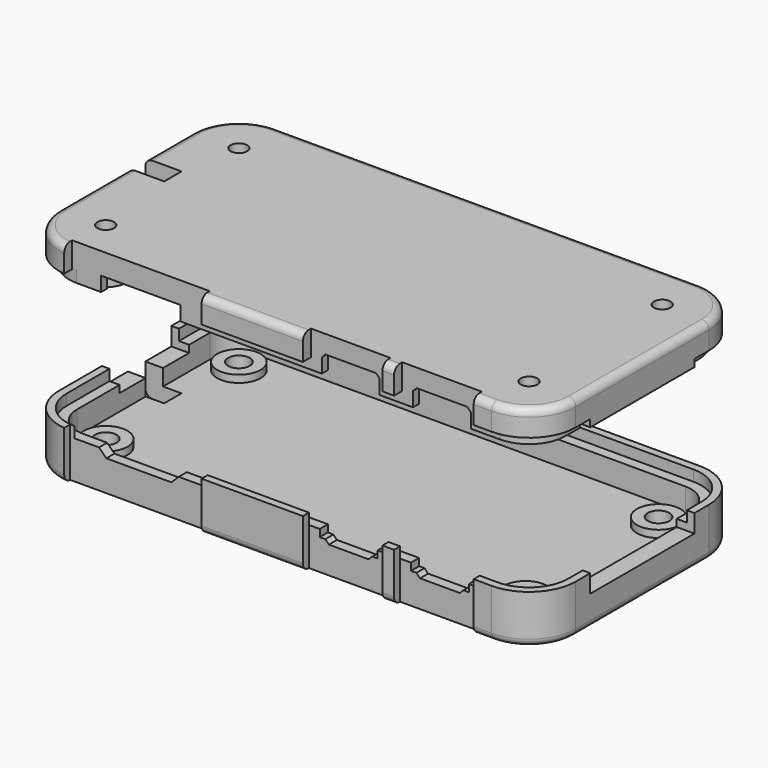
from build123d import *

# Parameters (mm, degrees)
F1_DEPTH  = 2
F2_DEPTH  = 3.25
F3_R      = 3
F4_DEPTH  = 1
F6_W      = 2.45
F6_H      = 12
F6_W_2    = 11
F6_H_2    = 2.45
F6_W_3    = 8
F6_H_3    = 18
F7_DEPTH  = 1
F10_DEPTH = 2
F11_DEPTH = 3
F12_W     = 2.45
F12_H     = 12
F13_DEPTH = 1
F12_W_2   = 11
F12_H_2   = 2.45
F14_DEPTH = 2
F12_W_3   = 8
F15_DEPTH = 2
F12_H_3   = 18
F16_DEPTH = 0.5
F17_R     = 3
F18_DEPTH = 4
F20_D     = 2.3
F20_DEPTH = 13
F20_TIP   = 0.6909897119
F22_D     = 3
F22_DEPTH = 13
F22_TIP   = 0.9012909285
F23_W     = 3
F23_H     = 4.25
F24_DEPTH = 5
F25_W     = 3
F25_H     = 4
F26_DEPTH = 5
F27_R     = 1
F27_2_R   = 1
F28_W     = 5.5
F28_H     = 2.45
F29_DEPTH = 0.5
F30_SIZE  = 0.49999
F31_W     = 7
F31_H     = 2.45
F32_DEPTH = 0.5
F33_SIZE  = 0.49999
F34_W     = 19.5
F34_H     = 1.4
F34_W_2   = 4.6
F35_DEPTH = 1.5
F37_W     = 4.6
F37_H     = 1.05
F37_W_2   = 19.5
F38_DEPTH = 1.5
F39_SIZE  = 1
F40_W     = 11
F40_H     = 3.5
F40_W_2   = 19
F41_DEPTH = 1.4
F42_W     = 11
F42_H     = 6.75
F42_W_2   = 19
F43_DEPTH = 1.05


# Not quite as in the source:
# - a fillet or chamfer is up to 0.001 mm smaller than in the source, because OpenCascade refuses the exact size


with BuildPart() as f1:
    # F0 (on Top) → F1 (new body)
    with BuildSketch(Plane.XY):
        with BuildLine():
            Line((62, 32.95), (3.5, 32.95))
            ThreePointArc((3.5, 32.95), (-1.0608387387, 31.0608387387), (-2.95, 26.5))
            Line((-2.95, 26.5), (-2.95, 3.5))
            ThreePointArc((-2.95, 3.5), (-1.0608387387, -1.0608387387), (3.5, -2.95))
            Line((3.5, -2.95), (62, -2.95))
            ThreePointArc((62, -2.95), (66.5608387387, -1.0608387387), (68.45, 3.5))
            Line((68.45, 3.5), (68.45, 26.5))
            ThreePointArc((68.45, 26.5), (66.5608387387, 31.0608387387), (62, 32.95))
        make_face()
        with BuildLine():
            ThreePointArc((-0.5, 26.5), (0.6715728753, 29.3284271247), (3.5, 30.5))
            Line((3.5, 30.5), (62, 30.5))
            ThreePointArc((62, 30.5), (64.8284271247, 29.3284271247), (66, 26.5))
            Line((66, 26.5), (66, 3.5))
            ThreePointArc((66, 3.5), (64.8284271247, 0.6715728753), (62, -0.5))
            Line((62, -0.5), (3.5, -0.5))
            ThreePointArc((3.5, -0.5), (0.6715728753, 0.6715728753), (-0.5, 3.5))
            Line((-0.5, 3.5), (-0.5, 26.5))
        make_face(mode=Mode.SUBTRACT)
        with BuildLine():
            Line((62, 30.5), (3.5, 30.5))
            ThreePointArc((3.5, 30.5), (0.6715728753, 29.3284271247), (-0.5, 26.5))
            Line((-0.5, 26.5), (-0.5, 3.5))
            ThreePointArc((-0.5, 3.5), (0.6715728753, 0.6715728753), (3.5, -0.5))
            Line((3.5, -0.5), (62, -0.5))
            ThreePointArc((62, -0.5), (64.8284271247, 0.6715728753), (66, 3.5))
            Line((66, 3.5), (66, 26.5))
            ThreePointArc((66, 26.5), (64.8284271247, 29.3284271247), (62, 30.5))
        make_face()
    extrude(amount=-F1_DEPTH)

    # F0 (on Top) → F2 (join)
    with BuildSketch(Plane.XY):
        with BuildLine():
            Line((62, 32.95), (3.5, 32.95))
            ThreePointArc((3.5, 32.95), (-1.0608387387, 31.0608387387), (-2.95, 26.5))
            Line((-2.95, 26.5), (-2.95, 3.5))
            ThreePointArc((-2.95, 3.5), (-1.0608387387, -1.0608387387), (3.5, -2.95))
            Line((3.5, -2.95), (62, -2.95))
            ThreePointArc((62, -2.95), (66.5608387387, -1.0608387387), (68.45, 3.5))
            Line((68.45, 3.5), (68.45, 26.5))
            ThreePointArc((68.45, 26.5), (66.5608387387, 31.0608387387), (62, 32.95))
        make_face()
        with BuildLine():
            ThreePointArc((-0.5, 26.5), (0.6715728753, 29.3284271247), (3.5, 30.5))
            Line((3.5, 30.5), (62, 30.5))
            ThreePointArc((62, 30.5), (64.8284271247, 29.3284271247), (66, 26.5))
            Line((66, 26.5), (66, 3.5))
            ThreePointArc((66, 3.5), (64.8284271247, 0.6715728753), (62, -0.5))
            Line((62, -0.5), (3.5, -0.5))
            ThreePointArc((3.5, -0.5), (0.6715728753, 0.6715728753), (-0.5, 3.5))
            Line((-0.5, 3.5), (-0.5, 26.5))
        make_face(mode=Mode.SUBTRACT)
    extrude(amount=F2_DEPTH)

    # F3 (on face) → F4 (join)
    with BuildSketch(Plane.XY):
        with Locations((3.5, 26.5)):
            Circle(F3_R)
        with Locations((61.5, 26.5)):
            Circle(F3_R)
        with Locations((61.5, 3.5)):
            Circle(F3_R)
        with Locations((3.5, 3.5)):
            Circle(F3_R)
    extrude(amount=F4_DEPTH)

    # F6 (on offset) → F7 (cut, through all)
    with BuildSketch(Plane.XY.offset(2.25)):
        with Locations((-1.725, 16.9)):
            Rectangle(F6_W, F6_H)
        with Locations((12.4, -1.725)):
            Rectangle(F6_W_2, F6_H_2)
        with Locations((41.4, -1.725)):
            Rectangle(F6_W_3, F6_H_2)
        with Locations((54, -1.725)):
            Rectangle(F6_W_3, F6_H_2)
        with Locations((67.225, 15)):
            Rectangle(F6_W, F6_H_3)
    extrude(amount=F7_DEPTH, mode=Mode.SUBTRACT)

    # F22
    with Locations(Plane.XY.offset(1)):
        with Locations((61.5, 26.5), (61.5, 3.5), (3.5, 3.5), (3.5, 26.5)):
            Hole(F22_D / 2, depth=F22_DEPTH)
            with Locations((0, 0, -(F22_DEPTH + F22_TIP / 2))):  # 118° drill point
                Cone(0, F22_D / 2, F22_TIP, mode=Mode.SUBTRACT)

    # F23 (on face) → F24 (cut)
    with BuildSketch(Plane(origin=(-2.95, 0, 0), x_dir=(0, -1, 0), z_dir=(-1, 0, 0))):
        with Locations((-16.9, 0.125)):
            Rectangle(F23_W, F23_H)
    extrude(amount=-F24_DEPTH, mode=Mode.SUBTRACT)

    # F27#2
    f27_2_edges = [f1.edges().sort_by_distance(p)[0] for p in [
        (66.560839, -1.060839, -2),
    ]]
    fillet(f27_2_edges, radius=F27_2_R)

    # F28 (on face) → F29 (cut)
    with BuildSketch(Plane.XY.offset(2.25)):
        with Locations((41.4, -1.725)):
            Rectangle(F28_W, F28_H)
        with Locations((54, -1.725)):
            Rectangle(F28_W, F28_H)
    extrude(amount=-F29_DEPTH, mode=Mode.SUBTRACT)

    # F30 (size 0.5 in the source; OpenCascade refuses exactly that, so slightly less here)
    f30_edges = [f1.edges().sort_by_distance(p)[0] for p in [
        (44.15, -1.725, 2.25),
        (38.65, -1.725, 2.25),
        (51.25, -1.725, 2.25),
        (56.75, -1.725, 2.25),
    ]]
    chamfer(f30_edges, length=F30_SIZE)

    # F37 (on face) → F38 (join)
    with BuildSketch(Plane.XY.offset(3.25)):
        with BuildLine():
            Line((68.45, 3.5), (68.45, 6))
            Line((68.45, 6), (67.4, 6))
            Line((67.4, 6), (67.4, 3.5))
            ThreePointArc((67.4, 3.5), (65.8183766184, -0.3183766184), (62, -1.9))
            Line((62, -1.9), (58, -1.9))
            Line((58, -1.9), (58, -2.95))
            Line((58, -2.95), (62, -2.95))
            ThreePointArc((62, -2.95), (66.5608387387, -1.0608387387), (68.45, 3.5))
        make_face()
        with Locations((47.7, -2.425)):
            Rectangle(F37_W, F37_H)
        with Locations((27.65, -2.425)):
            Rectangle(F37_W_2, F37_H)
        with BuildLine():
            ThreePointArc((-2.95, 3.5), (-1.0608387387, -1.0608387387), (3.5, -2.95))
            Line((3.5, -2.95), (6.9, -2.95))
            Line((6.9, -2.95), (6.9, -1.9))
            Line((6.9, -1.9), (3.5, -1.9))
            ThreePointArc((3.5, -1.9), (-0.3183766184, -0.3183766184), (-1.9, 3.5))
            Line((-1.9, 3.5), (-1.9, 10.9))
            Line((-1.9, 10.9), (-2.95, 10.9))
            Line((-2.95, 10.9), (-2.95, 3.5))
        make_face()
        with BuildLine():
            ThreePointArc((3.5, 32.95), (-1.0608387387, 31.0608387387), (-2.95, 26.5))
            Line((-2.95, 26.5), (-2.95, 22.9))
            Line((-2.95, 22.9), (-1.9, 22.9))
            Line((-1.9, 22.9), (-1.9, 26.5))
            ThreePointArc((-1.9, 26.5), (-0.3183766184, 30.3183766184), (3.5, 31.9))
            Line((3.5, 31.9), (62, 31.9))
            ThreePointArc((62, 31.9), (65.8183766184, 30.3183766184), (67.4, 26.5))
            Line((67.4, 26.5), (67.4, 24))
            Line((67.4, 24), (68.45, 24))
            Line((68.45, 24), (68.45, 26.5))
            ThreePointArc((68.45, 26.5), (66.5608387387, 31.0608387387), (62, 32.95))
            Line((62, 32.95), (3.5, 32.95))
        make_face()
    extrude(amount=F38_DEPTH)

    # F39
    f39_edges = [f1.edges().sort_by_distance(p)[0] for p in [
        (17.9, -1.725, 2.25),
        (6.9, -1.725, 2.25),
    ]]
    chamfer(f39_edges, length=F39_SIZE)

    # F42 (on face) → F43 (cut, through all)
    with BuildSketch(Plane.XZ.offset(2.95)):
        with Locations((54, 1.375)):
            Rectangle(F42_W, F42_H)
        with Locations((41.4, 1.375)):
            Rectangle(F42_W, F42_H)
        with Locations((12.4, 1.375)):
            Rectangle(F42_W_2, F42_H)
    extrude(amount=-F43_DEPTH, mode=Mode.SUBTRACT)


with BuildPart() as f10:
    # F9 (on offset) → F10 (new body)
    with BuildSketch(Plane.XY.offset(25)):
        with BuildLine():
            Line((62, 32.95), (3.5, 32.95))
            ThreePointArc((3.5, 32.95), (-1.0608387387, 31.0608387387), (-2.95, 26.5))
            Line((-2.95, 26.5), (-2.95, 3.5))
            ThreePointArc((-2.95, 3.5), (-1.0608387387, -1.0608387387), (3.5, -2.95))
            Line((3.5, -2.95), (62, -2.95))
            ThreePointArc((62, -2.95), (66.5608387387, -1.0608387387), (68.45, 3.5))
            Line((68.45, 3.5), (68.45, 26.5))
            ThreePointArc((68.45, 26.5), (66.5608387387, 31.0608387387), (62, 32.95))
        make_face()
        with BuildLine():
            Line((62, -0.5), (3.5, -0.5))
            ThreePointArc((3.5, -0.5), (0.6715728753, 0.6715728753), (-0.5, 3.5))
            Line((-0.5, 3.5), (-0.5, 26.5))
            ThreePointArc((-0.5, 26.5), (0.6715728753, 29.3284271247), (3.5, 30.5))
            Line((3.5, 30.5), (62, 30.5))
            ThreePointArc((62, 30.5), (64.8284271247, 29.3284271247), (66, 26.5))
            Line((66, 26.5), (66, 3.5))
            ThreePointArc((66, 3.5), (64.8284271247, 0.6715728753), (62, -0.5))
        make_face(mode=Mode.SUBTRACT)
        with BuildLine():
            ThreePointArc((-0.5, 3.5), (0.6715728753, 0.6715728753), (3.5, -0.5))
            Line((3.5, -0.5), (62, -0.5))
            ThreePointArc((62, -0.5), (64.8284271247, 0.6715728753), (66, 3.5))
            Line((66, 3.5), (66, 26.5))
            ThreePointArc((66, 26.5), (64.8284271247, 29.3284271247), (62, 30.5))
            Line((62, 30.5), (3.5, 30.5))
            ThreePointArc((3.5, 30.5), (0.6715728753, 29.3284271247), (-0.5, 26.5))
            Line((-0.5, 26.5), (-0.5, 3.5))
        make_face()
    extrude(amount=F10_DEPTH)

    # F9 (on offset) → F11 (join)
    with BuildSketch(Plane.XY.offset(25)):
        with BuildLine():
            Line((62, 32.95), (3.5, 32.95))
            ThreePointArc((3.5, 32.95), (-1.0608387387, 31.0608387387), (-2.95, 26.5))
            Line((-2.95, 26.5), (-2.95, 3.5))
            ThreePointArc((-2.95, 3.5), (-1.0608387387, -1.0608387387), (3.5, -2.95))
            Line((3.5, -2.95), (62, -2.95))
            ThreePointArc((62, -2.95), (66.5608387387, -1.0608387387), (68.45, 3.5))
            Line((68.45, 3.5), (68.45, 26.5))
            ThreePointArc((68.45, 26.5), (66.5608387387, 31.0608387387), (62, 32.95))
        make_face()
        with BuildLine():
            Line((62, -0.5), (3.5, -0.5))
            ThreePointArc((3.5, -0.5), (0.6715728753, 0.6715728753), (-0.5, 3.5))
            Line((-0.5, 3.5), (-0.5, 26.5))
            ThreePointArc((-0.5, 26.5), (0.6715728753, 29.3284271247), (3.5, 30.5))
            Line((3.5, 30.5), (62, 30.5))
            ThreePointArc((62, 30.5), (64.8284271247, 29.3284271247), (66, 26.5))
            Line((66, 26.5), (66, 3.5))
            ThreePointArc((66, 3.5), (64.8284271247, 0.6715728753), (62, -0.5))
        make_face(mode=Mode.SUBTRACT)
    extrude(amount=-F11_DEPTH)

    # F12 (on face) → F13 (cut)
    with BuildSketch(Plane(origin=(0, 0, 22), x_dir=(1, 0, 0), z_dir=(0, 0, -1))):
        with Locations((-1.725, -16.9)):
            Rectangle(F12_W, F12_H)
    extrude(amount=-F13_DEPTH, mode=Mode.SUBTRACT)

    # F12 (on face) → F14 (cut)
    with BuildSketch(Plane(origin=(0, 0, 22), x_dir=(1, 0, 0), z_dir=(0, 0, -1))):
        with Locations((12.4, 1.725)):
            Rectangle(F12_W_2, F12_H_2)
    extrude(amount=-F14_DEPTH, mode=Mode.SUBTRACT)

    # F12 (on face) → F15 (cut)
    with BuildSketch(Plane(origin=(0, 0, 22), x_dir=(1, 0, 0), z_dir=(0, 0, -1))):
        with Locations((41.4, 1.725)):
            Rectangle(F12_W_3, F12_H_2)
        with Locations((54, 1.725)):
            Rectangle(F12_W_3, F12_H_2)
    extrude(amount=-F15_DEPTH, mode=Mode.SUBTRACT)

    # F12 (on face) → F16 (cut)
    with BuildSketch(Plane(origin=(0, 0, 22), x_dir=(1, 0, 0), z_dir=(0, 0, -1))):
        with Locations((67.225, -15)):
            Rectangle(F12_W, F12_H_3)
    extrude(amount=-F16_DEPTH, mode=Mode.SUBTRACT)

    # F17 (on offset) → F18 (join)
    with BuildSketch(Plane.XY.offset(25)):
        with Locations((3.5, 26.5)):
            Circle(F17_R)
        with Locations((3.5, 3.5)):
            Circle(F17_R)
        with Locations((62, 3.5)):
            Circle(F17_R)
        with Locations((62, 26.5)):
            Circle(F17_R)
    extrude(amount=-F18_DEPTH)

    # F20
    with Locations(Plane(origin=(0, 0, 21), x_dir=(1, 0, 0), z_dir=(0, 0, -1))):
        with Locations((62, -26.5), (62, -3.5), (3.5, -3.5), (3.5, -26.5)):
            Hole(F20_D / 2, depth=F20_DEPTH)
            with Locations((0, 0, -(F20_DEPTH + F20_TIP / 2))):  # 118° drill point
                Cone(0, F20_D / 2, F20_TIP, mode=Mode.SUBTRACT)

    # F25 (on face) → F26 (cut)
    with BuildSketch(Plane(origin=(-2.95, 0, 0), x_dir=(0, -1, 0), z_dir=(-1, 0, 0))):
        with Locations((-16.9, 25)):
            Rectangle(F25_W, F25_H)
    extrude(amount=-F26_DEPTH, mode=Mode.SUBTRACT)

    # F27
    f27_edges = [f10.edges().sort_by_distance(p)[0] for p in [
        (32.75, -2.95, 27),
    ]]
    fillet(f27_edges, radius=F27_R)

    # F31 (on face) → F32 (cut)
    with BuildSketch(Plane(origin=(0, 0, 24), x_dir=(1, 0, 0), z_dir=(0, 0, -1))):
        with Locations((41.4, 1.725)):
            Rectangle(F31_W, F31_H)
        with Locations((54, 1.725)):
            Rectangle(F31_W, F31_H)
    extrude(amount=-F32_DEPTH, mode=Mode.SUBTRACT)

    # F33 (size 0.5 in the source; OpenCascade refuses exactly that, so slightly less here)
    f33_edges = [f10.edges().sort_by_distance(p)[0] for p in [
        (44.9, -1.725, 24),
        (57.5, -1.725, 24),
        (50.5, -1.725, 24),
        (37.9, -1.725, 24),
    ]]
    chamfer(f33_edges, length=F33_SIZE)

    # F34 (on face) → F35 (cut)
    with BuildSketch(Plane(origin=(0, 0, 22), x_dir=(1, 0, 0), z_dir=(0, 0, -1))):
        with BuildLine():
            ThreePointArc((-1.55, -3.5), (-0.070889245, 0.070889245), (3.5, 1.55))
            Line((3.5, 1.55), (6.9, 1.55))
            Line((6.9, 1.55), (6.9, 2.95))
            Line((6.9, 2.95), (3.5, 2.95))
            ThreePointArc((3.5, 2.95), (-1.0608387387, 1.0608387387), (-2.95, -3.5))
            Line((-2.95, -3.5), (-2.95, -10.9))
            Line((-2.95, -10.9), (-1.55, -10.9))
            Line((-1.55, -10.9), (-1.55, -3.5))
        make_face()
        with Locations((27.65, 2.25)):
            Rectangle(F34_W, F34_H)
        with Locations((47.7, 2.25)):
            Rectangle(F34_W_2, F34_H)
        with BuildLine():
            Line((67.05, -3.5), (67.05, -6))
            Line((67.05, -6), (68.45, -6))
            Line((68.45, -6), (68.45, -3.5))
            ThreePointArc((68.45, -3.5), (66.5608387387, 1.0608387387), (62, 2.95))
            Line((62, 2.95), (58, 2.95))
            Line((58, 2.95), (58, 1.55))
            Line((58, 1.55), (62, 1.55))
            ThreePointArc((62, 1.55), (65.570889245, 0.070889245), (67.05, -3.5))
        make_face()
        with BuildLine():
            Line((67.05, -24), (67.05, -26.5))
            ThreePointArc((67.05, -26.5), (65.570889245, -30.070889245), (62, -31.55))
            Line((62, -31.55), (3.5, -31.55))
            ThreePointArc((3.5, -31.55), (-0.070889245, -30.070889245), (-1.55, -26.5))
            Line((-1.55, -26.5), (-1.55, -22.9))
            Line((-1.55, -22.9), (-2.95, -22.9))
            Line((-2.95, -22.9), (-2.95, -26.5))
            ThreePointArc((-2.95, -26.5), (-1.0608387387, -31.0608387387), (3.5, -32.95))
            Line((3.5, -32.95), (62, -32.95))
            ThreePointArc((62, -32.95), (66.5608387387, -31.0608387387), (68.45, -26.5))
            Line((68.45, -26.5), (68.45, -24))
            Line((68.45, -24), (67.05, -24))
        make_face()
    extrude(amount=-F35_DEPTH, mode=Mode.SUBTRACT)

    # F40 (on face) → F41 (cut, through all)
    with BuildSketch(Plane.XZ.offset(2.95)):
        with Locations((41.4, 25.25)):
            Rectangle(F40_W, F40_H)
        with Locations((54, 25.25)):
            Rectangle(F40_W, F40_H)
        with Locations((12.4, 25.25)):
            Rectangle(F40_W_2, F40_H)
    extrude(amount=-F41_DEPTH, mode=Mode.SUBTRACT)


solid = Compound([f1.part, f10.part])
